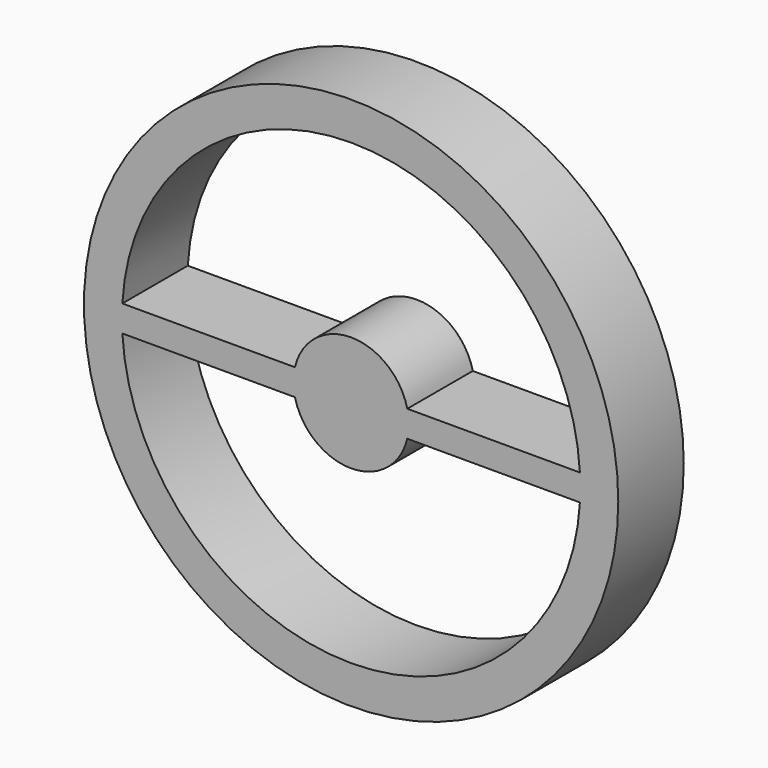
from build123d import *

# Parameters (mm, degrees)
F0_R     = 10.3601879012
F1_DEPTH = 3.175
F2_R     = 10.3601879012
F3_DEPTH = 3.175


with BuildPart() as f1:
    # F0 (on Front) → F1 (new body)
    with BuildSketch(Plane.XZ):
        Circle(F0_R)
        with BuildLine():
            ThreePointArc((9.5114533333, 0.5078193457), (9.521612731, 0.254), (9.525, 0))
            ThreePointArc((9.525, 0), (9.5215246826, -0.2572794566), (9.5111012664, -0.5143711699))
            ThreePointArc((9.5111012664, -0.5143711699), (0, -9.525), (-9.5111012664, -0.5143711699))
            ThreePointArc((-9.5111012664, -0.5143711699), (-9.524999435, -0.0032806383), (-9.5114533333, 0.5078193457))
            ThreePointArc((-9.5114533333, 0.5078193457), (0, 9.525), (9.5114533333, 0.5078193457))
        make_face(mode=Mode.SUBTRACT)
        with BuildLine():
            Line((-2.1784585047, 0.5078193457), (-9.5114533333, 0.5078193457))
            ThreePointArc((-9.5114533333, 0.5078193457), (-9.524999435, -0.0032806383), (-9.5111012664, -0.5143711699))
            Line((-9.5111012664, -0.5143711699), (-2.1769208171, -0.5143711699))
            ThreePointArc((-2.1769208171, -0.5143711699), (-2.2368617797, -0.0033649251), (-2.1784585047, 0.5078193457))
        make_face()
        with BuildLine():
            ThreePointArc((2.2368643107, 0), (2.222214889, 0.2555835118), (2.1784585047, 0.5078193457))
            ThreePointArc((2.1784585047, 0.5078193457), (0, 2.2368643107), (-2.1784585047, 0.5078193457))
            ThreePointArc((-2.1784585047, 0.5078193457), (-2.2368617797, -0.0033649251), (-2.1769208171, -0.5143711699))
            ThreePointArc((-2.1769208171, -0.5143711699), (0, -2.2368643107), (2.1769208171, -0.5143711699))
            ThreePointArc((2.1769208171, -0.5143711699), (2.2218278992, -0.2589261105), (2.2368643107, 0))
        make_face()
        with BuildLine():
            ThreePointArc((9.5111012664, -0.5143711699), (9.5215246826, -0.2572794566), (9.525, 0))
            ThreePointArc((9.525, 0), (9.521612731, 0.254), (9.5114533333, 0.5078193457))
            Line((9.5114533333, 0.5078193457), (2.1784585047, 0.5078193457))
            ThreePointArc((2.1784585047, 0.5078193457), (2.222214889, 0.2555835118), (2.2368643107, 0))
            ThreePointArc((2.2368643107, 0), (2.2218278992, -0.2589261105), (2.1769208171, -0.5143711699))
            Line((2.1769208171, -0.5143711699), (9.5111012664, -0.5143711699))
        make_face()
    extrude(amount=F1_DEPTH)

    # F2 (on face) → F3 (join)
    with BuildSketch(Plane.XZ.offset(3.175)):
        Circle(F2_R)
        with BuildLine():
            ThreePointArc((8.8731253784, 0.5078193457), (8.8840143878, 0.2540134389), (8.8876450463, 0))
            ThreePointArc((8.8876450463, 0), (8.8839199998, -0.2572934234), (8.872747983, -0.5143711699))
            Line((8.872747983, -0.5143711699), (9.5111012664, -0.5143711699))
            ThreePointArc((9.5111012664, -0.5143711699), (0, -9.525), (-9.5111012664, -0.5143711699))
            Line((-9.5111012664, -0.5143711699), (-8.872747983, -0.5143711699))
            ThreePointArc((-8.872747983, -0.5143711699), (-8.8876444406, -0.0032813423), (-8.8731253784, 0.5078193457))
            Line((-8.8731253784, 0.5078193457), (-9.5114533333, 0.5078193457))
            ThreePointArc((-9.5114533333, 0.5078193457), (0, 9.525), (9.5114533333, 0.5078193457))
            Line((9.5114533333, 0.5078193457), (8.8731253784, 0.5078193457))
        make_face(mode=Mode.SUBTRACT)
        with BuildLine():
            ThreePointArc((-8.8731253784, 0.5078193457), (0, 8.8876450463), (8.8731253784, 0.5078193457))
            Line((8.8731253784, 0.5078193457), (9.5114533333, 0.5078193457))
            ThreePointArc((9.5114533333, 0.5078193457), (0, 9.525), (-9.5114533333, 0.5078193457))
            Line((-9.5114533333, 0.5078193457), (-8.8731253784, 0.5078193457))
        make_face()
        with BuildLine():
            Line((9.5111012664, -0.5143711699), (8.872747983, -0.5143711699))
            ThreePointArc((8.872747983, -0.5143711699), (0, -8.8876450463), (-8.872747983, -0.5143711699))
            Line((-8.872747983, -0.5143711699), (-9.5111012664, -0.5143711699))
            ThreePointArc((-9.5111012664, -0.5143711699), (0, -9.525), (9.5111012664, -0.5143711699))
        make_face()
    extrude(amount=-F3_DEPTH)


solid = f1.part
